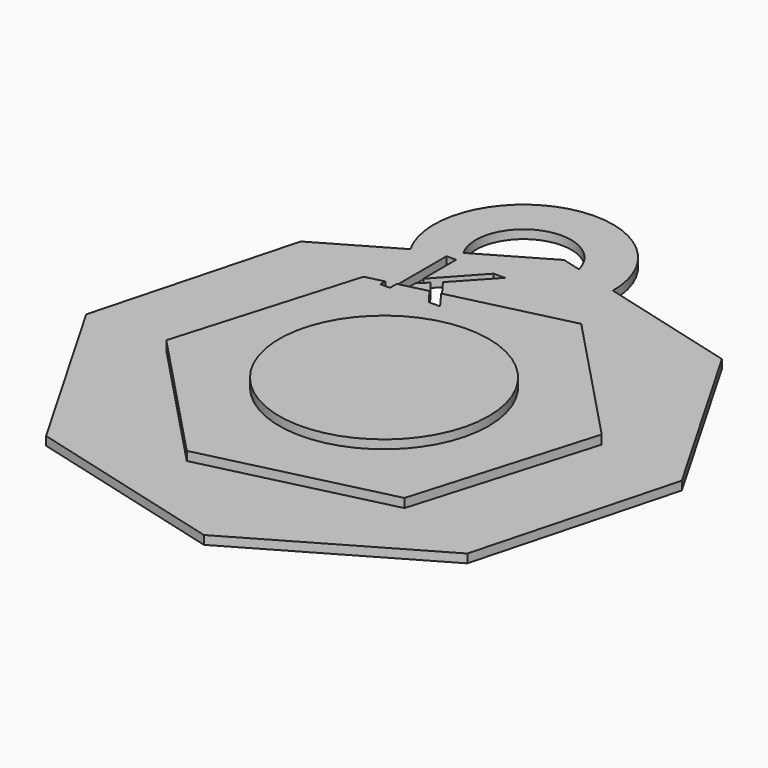
from build123d import *

# Parameters (mm, degrees)
F1_DEPTH     = 2
F3_DEPTH     = 4.064
F4_R         = 24.1844327061
F5_DEPTH     = 2
F6_R         = 20.6696582535
F6_R_2       = 11.012816468
F7_DEPTH     = 2
F8_TEXT_SIZE = 26.7619862118
F9_DEPTH     = 25.4


# Not quite as in the source:
# - Text() gives the source's letters only with a copy of the font that has no kerning and outlines rounded to 1/6400 em; it was checked with that copy


with BuildPart() as f1:
    # F0 (on Top) → F1 (new body)
    with BuildSketch(Plane.XY):
        Polygon((8.1930972305, -62.2297780189), (49.7964926395, -38.2097034183), (62.2297780189, 8.1930972305), (38.2097034183, 49.7964926395), (-8.1930972305, 62.2297780189), (-49.7964926395, 38.2097034183), (-62.2297780189, -8.1930972305), (-38.2097034183, -49.7964926395), align=None)
    extrude(amount=F1_DEPTH)

    # F2 (on face) → F3 (join)
    with BuildSketch(Plane(origin=(0, 0, 0), x_dir=(1, 0, 0), z_dir=(0, 0, -1))):
        Polygon((29.8738798744, 31.4332983472), (-12.2850949562, 41.5881880544), (-42.1589748306, 10.1548897072), (-29.8738798744, -31.4332983472), (12.2850949562, -41.5881880544), (42.1589748306, -10.1548897072), align=None)
    extrude(amount=-F3_DEPTH)

    # F4 (on face) → F5 (join)
    with BuildSketch(Plane.XY.offset(4.064)):
        Circle(F4_R)
    extrude(amount=F5_DEPTH)

    # F6 (on Top) → F7 (join)
    with BuildSketch(Plane.XY):
        with Locations((-14.5106706768, 58.4180727601)):
            Circle(F6_R)
        with Locations((-14.5106706768, 58.4180727601)):
            Circle(F6_R_2, mode=Mode.SUBTRACT)
    extrude(amount=F7_DEPTH)

    # F8 (on face) → F9 (cut)
    with BuildSketch(Plane.XY.offset(6.064)):
        with Locations((-28.2884724438, 31.0241039842)):
            Text('K', F8_TEXT_SIZE, font='Open Sans', text_align=(TextAlign.LEFT, TextAlign.BOTTOM))
    extrude(amount=-F9_DEPTH, mode=Mode.SUBTRACT)


solid = f1.part
